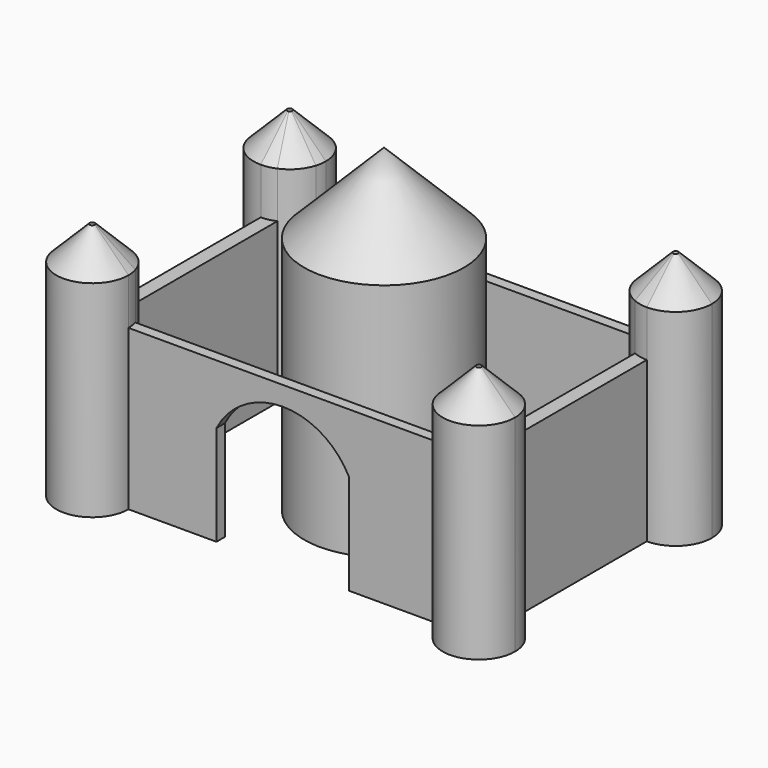
from build123d import *

# Parameters (mm, degrees)
F1_DEPTH  = 25.4
F2_DEPTH  = 38.1
F0_R      = 12.7
F3_DEPTH  = 50.8
F5_DEPTH  = 25.4
F6_SIZE   = 12.7
F7_SIZE   = 5.334
F7_2_SIZE = 5.334
F7_3_SIZE = 5.334
F7_4_SIZE = 5.334


# Not quite as in the source:
# - a feature names something its author has since deleted; it is built from what else it names


with BuildPart() as f1:
    # F0 (on Top) → F1 (new body)
    with BuildSketch(Plane.XY):
        with BuildLine():
            Line((24.9506174104, 19.6146306736), (-24.950613876, 19.6146306736))
            ThreePointArc((-24.950613876, 19.6146306736), (-25.0127463025, 18.7718966911), (-25.1977999521, 17.9473870487))
            Line((-25.1977999521, 17.9473870487), (25.1978040222, 17.9473870487))
            ThreePointArc((25.1978040222, 17.9473870487), (25.0127501018, 18.771896671), (24.9506174104, 19.6146306736))
        make_face()
    extrude(amount=F1_DEPTH)


with BuildPart() as f1b:
    # F0 (on Top) → F1, piece 2 (new body)
    with BuildSketch(Plane.XY):
        with BuildLine():
            Line((-30.6968968099, 13.8683477398), (-30.6968968099, -13.8683477398))
            ThreePointArc((-30.6968968099, -13.8683477398), (-29.54571818, -13.9848389086), (-28.4412139466, -14.3295892948))
            Line((-28.4412139466, -14.3295892948), (-28.4412139466, 14.3295892948))
            ThreePointArc((-28.4412139466, 14.3295892948), (-29.54571818, 13.9848389086), (-30.6968968099, 13.8683477398))
        make_face()
    extrude(amount=F1_DEPTH)


with BuildPart() as f1c:
    # F0 (on Top) → F1, piece 3 (new body)
    with BuildSketch(Plane.XY):
        with BuildLine():
            ThreePointArc((-25.1977999521, -17.9473870487), (-25.0127463025, -18.7718966911), (-24.950613876, -19.6146306736))
            Line((-24.950613876, -19.6146306736), (24.9514508717, -19.6146306736))
            ThreePointArc((24.9514508717, -19.6146306736), (24.9989231754, -18.7730083224), (25.1690152512, -17.9473870487))
            Line((25.1690152512, -17.9473870487), (-25.1977999521, -17.9473870487))
        make_face()
    extrude(amount=F1_DEPTH)

    # F4 (on face) → F5 (cut)
    with BuildSketch(Plane.XZ.offset(19.6146306736)):
        with BuildLine():
            Line((-10.9574375674, 15.9193035215), (-10.9574375674, 0))
            Line((-10.9574375674, 0), (10.130468756, 0))
            Line((10.130468756, 0), (10.130468756, 15.9193035215))
            ThreePointArc((10.130468756, 15.9193035215), (-0.4134844057, 22.3445965305), (-10.9574375674, 15.9193035215))
        make_face()
    extrude(amount=-F5_DEPTH, mode=Mode.SUBTRACT)


with BuildPart() as f1d:
    # F0 (on Top) → F1, piece 4 (new body)
    with BuildSketch(Plane.XY):
        with BuildLine():
            Line((28.4412139466, 14.3295925704), (28.4412139466, -14.2315152048))
            ThreePointArc((28.4412139466, -14.2315152048), (29.54571818, -13.8867648186), (30.6968968099, -13.7702736498))
            Line((30.6968968099, -13.7702736498), (30.6968968099, 13.868349507))
            ThreePointArc((30.6968968099, 13.868349507), (29.5457181005, 13.9848414147), (28.4412139466, 14.3295925704))
        make_face()
    extrude(amount=F1_DEPTH)


with BuildPart() as f2:
    # F0 (on Top) → F2 (new body)
    with BuildSketch(Plane.XY):
        with BuildLine():
            ThreePointArc((-24.950613876, 19.6146306736), (-34.760132439, 23.6778663028), (-30.6968968099, 13.8683477398))
            ThreePointArc((-30.6968968099, 13.8683477398), (-29.54571818, 13.9848389086), (-28.4412139466, 14.3295892948))
            ThreePointArc((-28.4412139466, 14.3295892948), (-26.4183144188, 15.778812602), (-25.1977999521, 17.9473870487))
            ThreePointArc((-25.1977999521, 17.9473870487), (-25.0127463025, 18.7718966911), (-24.950613876, 19.6146306736))
        make_face()
    extrude(amount=F2_DEPTH)

    # F7
    f7_edges = [f2.edges().sort_by_distance(p)[0] for p in [
        (-30.696897, 25.360914, 38.1),
    ]]
    chamfer(f7_edges, length=F7_SIZE)


with BuildPart() as f2b:
    # F0 (on Top) → F2, piece 2 (new body)
    with BuildSketch(Plane.XY):
        with BuildLine():
            ThreePointArc((25.1978040222, 17.9473870487), (26.4183172869, 15.7788151124), (28.4412139466, 14.3295925704))
            ThreePointArc((28.4412139466, 14.3295925704), (29.5457181005, 13.9848414147), (30.6968968099, 13.868349507))
            ThreePointArc((30.6968968099, 13.868349507), (34.7601347238, 15.5513955621), (36.4431832781, 19.6146324408))
            ThreePointArc((36.4431832781, 19.6146324408), (30.6968994606, 25.3609153747), (24.9506174104, 19.6146306736))
            ThreePointArc((24.9506174104, 19.6146306736), (25.0127501018, 18.771896671), (25.1978040222, 17.9473870487))
        make_face()
    extrude(amount=F2_DEPTH)

    # F7#2
    f7_2_edges = [f2b.edges().sort_by_distance(p)[0] for p in [
        (36.443183, 19.614634, 38.1),
    ]]
    chamfer(f7_2_edges, length=F7_2_SIZE)


with BuildPart() as f2c:
    # F0 (on Top) → F2, piece 3 (new body)
    with BuildSketch(Plane.XY):
        with BuildLine():
            ThreePointArc((-30.6968968099, -13.8683477398), (-34.760132439, -23.6778663028), (-24.950613876, -19.6146306736))
            ThreePointArc((-24.950613876, -19.6146306736), (-25.0127463025, -18.7718966911), (-25.1977999521, -17.9473870487))
            ThreePointArc((-25.1977999521, -17.9473870487), (-26.4183144188, -15.778812602), (-28.4412139466, -14.3295892948))
            ThreePointArc((-28.4412139466, -14.3295892948), (-29.54571818, -13.9848389086), (-30.6968968099, -13.8683477398))
        make_face()
    extrude(amount=F2_DEPTH)

    # F7#3
    f7_3_edges = [f2c.edges().sort_by_distance(p)[0] for p in [
        (-36.44318, -19.614631, 38.1),
    ]]
    chamfer(f7_3_edges, length=F7_3_SIZE)


with BuildPart() as f2d:
    # F0 (on Top) → F2, piece 4 (new body)
    with BuildSketch(Plane.XY):
        with BuildLine():
            ThreePointArc((25.1690152512, -17.9473870487), (24.9989231754, -18.7730083224), (24.9514508717, -19.6146306736))
            ThreePointArc((24.9514508717, -19.6146306736), (30.7459356406, -25.2626302648), (36.4431797437, -19.5165565837))
            ThreePointArc((36.4431797437, -19.5165565837), (34.760132439, -15.4533209545), (30.6968968099, -13.7702736498))
            ThreePointArc((30.6968968099, -13.7702736498), (29.54571818, -13.8867648186), (28.4412139466, -14.2315152048))
            ThreePointArc((28.4412139466, -14.2315152048), (26.3843691674, -15.718942479), (25.1690152512, -17.9473870487))
        make_face()
    extrude(amount=F2_DEPTH)

    # F7#4
    f7_4_edges = [f2d.edges().sort_by_distance(p)[0] for p in [
        (36.442343, -19.418482, 38.1),
    ]]
    chamfer(f7_4_edges, length=F7_4_SIZE)


with BuildPart() as f3:
    # F0 (on Top) → F3 (new body)
    with BuildSketch(Plane.XY):
        Circle(F0_R)
    extrude(amount=F3_DEPTH)

    # F6
    f6_edges = [f3.edges().sort_by_distance(p)[0] for p in [
        (-12.7, 0, 50.8),
    ]]
    chamfer(f6_edges, length=F6_SIZE)


solid = Compound([f1.part, f1b.part, f1c.part, f1d.part, f2.part, f2b.part, f2c.part, f2d.part, f3.part])
